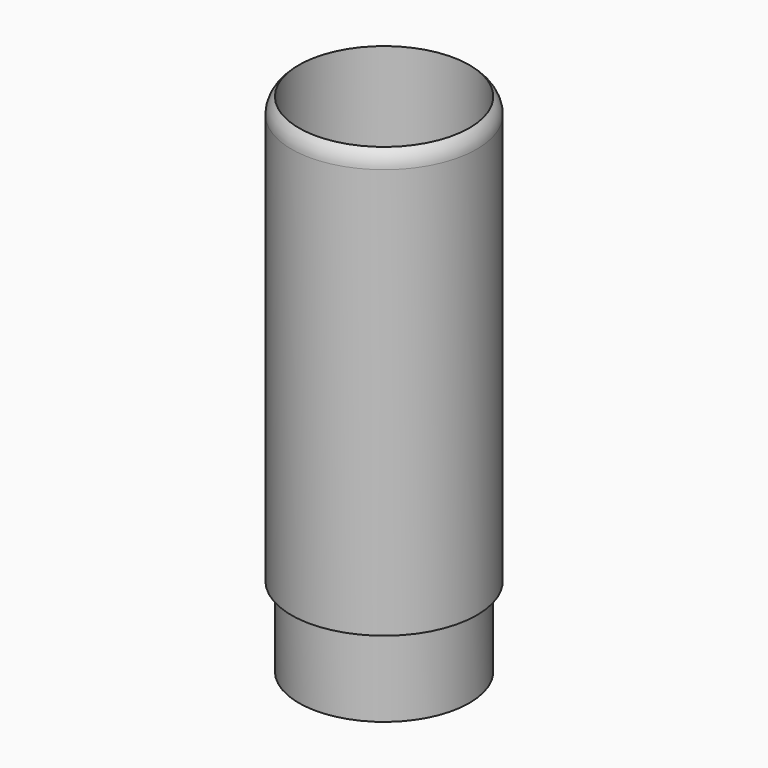
from build123d import *

# Parameters (mm, degrees)
F0_R     = 20
F1_DEPTH = 18.7
F2_R     = 21.75
F2_R_2   = 20
F3_DEPTH = 100
F4_R     = 17.5
F5_DEPTH = 25


# Not quite as in the source:
# - a fillet or chamfer that OpenCascade refuses, or shapes differently, is made with other operations: its cross-section is extruded or revolved along the edge and cut away or added


with BuildPart() as f1:
    # F0 (on Top) → F1 (new body)
    with BuildSketch(Plane.XY):
        Circle(F0_R)
    extrude(amount=F1_DEPTH)

    # F4 (on face) → F5 (cut)
    with BuildSketch(Plane.XY.offset(18.7)):
        Circle(F4_R)
    extrude(amount=-F5_DEPTH, mode=Mode.SUBTRACT)


with BuildPart() as f3:
    # F2 (on face) → F3 (new body)
    with BuildSketch(Plane.XY.offset(18.7)):
        Circle(F2_R)
        Circle(F2_R_2, mode=Mode.SUBTRACT)
    extrude(amount=F3_DEPTH)

    # F6: fillet of radius 5 on 1 edges, made by hand

    # F6_s1 → F6_t2 (revolve, cut)
    with BuildSketch(Plane.XZ):
        with BuildLine():
            ThreePointArc((21.75, 114.9003289616), (21.2914755311, 116.9919790279), (20, 118.7))
            Line((20, 118.7), (21.75, 118.7))
            Line((21.75, 118.7), (21.75, 114.9003289616))
        make_face()
    revolve(axis=Axis((0, 0, 118.7), (0, 0, 1)), mode=Mode.SUBTRACT)


solid = Compound([f1.part, f3.part])
